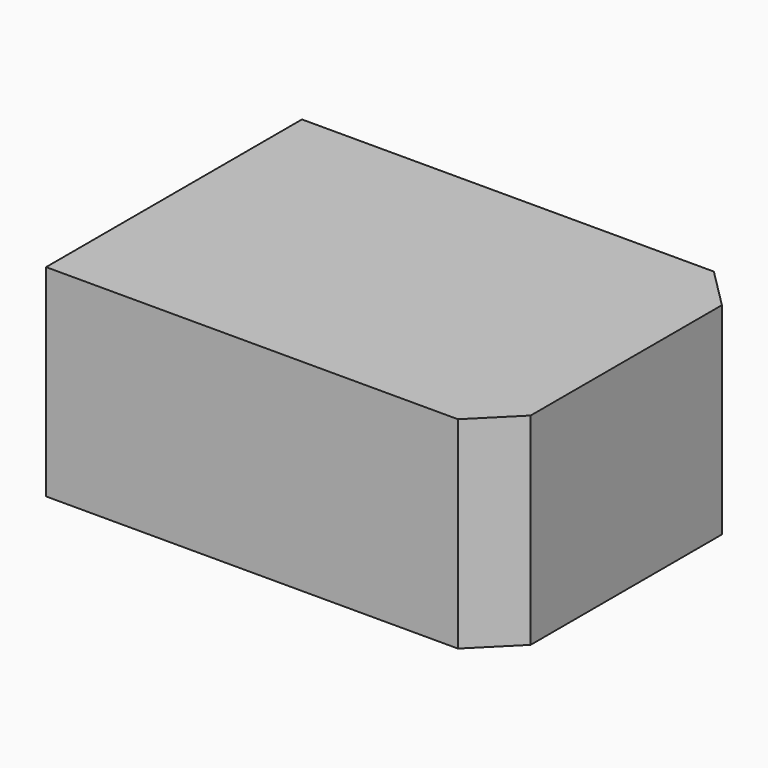
from build123d import *

# Parameters (mm, degrees)
F0_W     = 56.8971335888
F0_H     = 40.2365922928
F1_DEPTH = 25.4
F2_SIZE  = 5.08
F5_T     = -2.54


# Not quite as in the source:
# - the program builds the solid bodies; features that only make, move or delete a surface that nothing else refers to are left out


with BuildPart() as f1:
    # F0 (on Top) → F1 (new body)
    with BuildSketch(Plane.XY):
        with Locations((12.4524980783, -20.1182961464)):
            Rectangle(F0_W, F0_H)
    extrude(amount=F1_DEPTH)

    # F2
    f2_edges = [f1.edges().sort_by_distance(p)[0] for p in [
        (40.901065, -40.236592, 12.7),
        (40.901065, 0, 12.7),
    ]]
    chamfer(f2_edges, length=F2_SIZE)

    # F5
    f5_openings = [f1.faces().sort_by_distance(p)[0] for p in [
        (12.147464, -20.118296, 0),
    ]]
    offset(amount=F5_T, openings=f5_openings)


solid = f1.part
